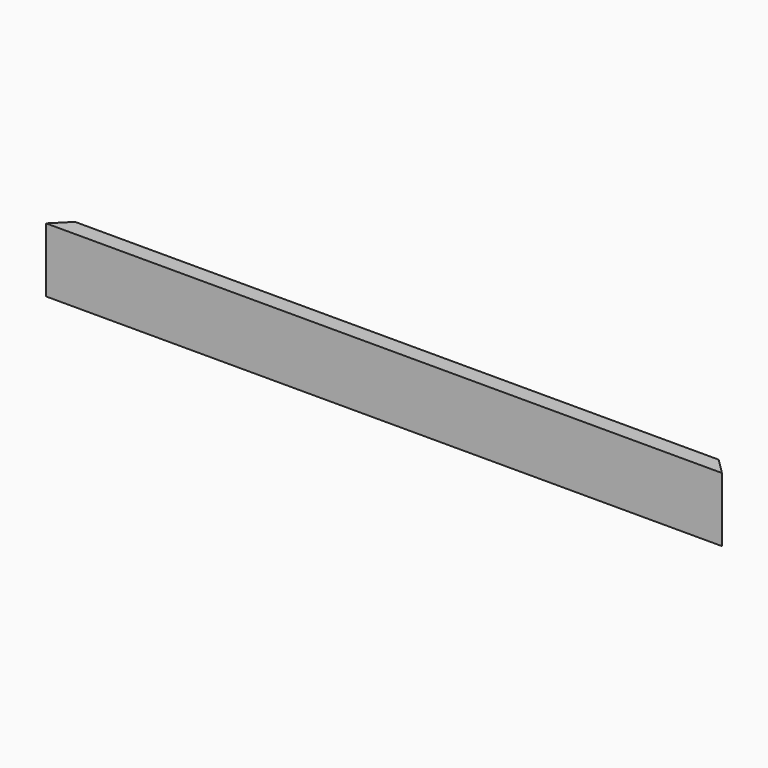
from build123d import *

# Parameters (mm, degrees)
F0_W        = 50.8
F0_H        = 203.2
F0_W_2      = 41.275
F0_H_2      = 193.675
F1_DEPTH    = 2133.6
F2_T1_DEPTH = 464.4829915773
F3_T1_DEPTH = 464.4829915773


# Not quite as in the source:
# - a fillet or chamfer that OpenCascade refuses, or shapes differently, is made with other operations: its cross-section is extruded or revolved along the edge and cut away or added


with BuildPart() as f1:
    # F0 (on Right) → F1 (new body)
    with BuildSketch(Plane.YZ):
        with Locations((25.4, 101.6)):
            Rectangle(F0_W, F0_H)
        with Locations((25.4, 101.6)):
            Rectangle(F0_W_2, F0_H_2, mode=Mode.SUBTRACT)
    extrude(amount=-F1_DEPTH)

    # F2: chamfer of 50.8 on 1 edges, made by hand

    # F2_s2 → F2_t1 (cut)
    with BuildSketch(Plane.XY.offset(-130.6414957887)):
        Polygon((-50.8, 50.8), (0, 0), (0, 50.8), align=None)
    extrude(amount=F2_T1_DEPTH, mode=Mode.SUBTRACT)

    # F3: chamfer of 50.8 on 1 edges, made by hand

    # F3_s2 → F3_t1 (cut)
    with BuildSketch(Plane.XY.offset(-130.6414957887)):
        Polygon((-2133.6, 0), (-2082.8, 50.8), (-2133.6, 50.8), align=None)
    extrude(amount=F3_T1_DEPTH, mode=Mode.SUBTRACT)


solid = f1.part
